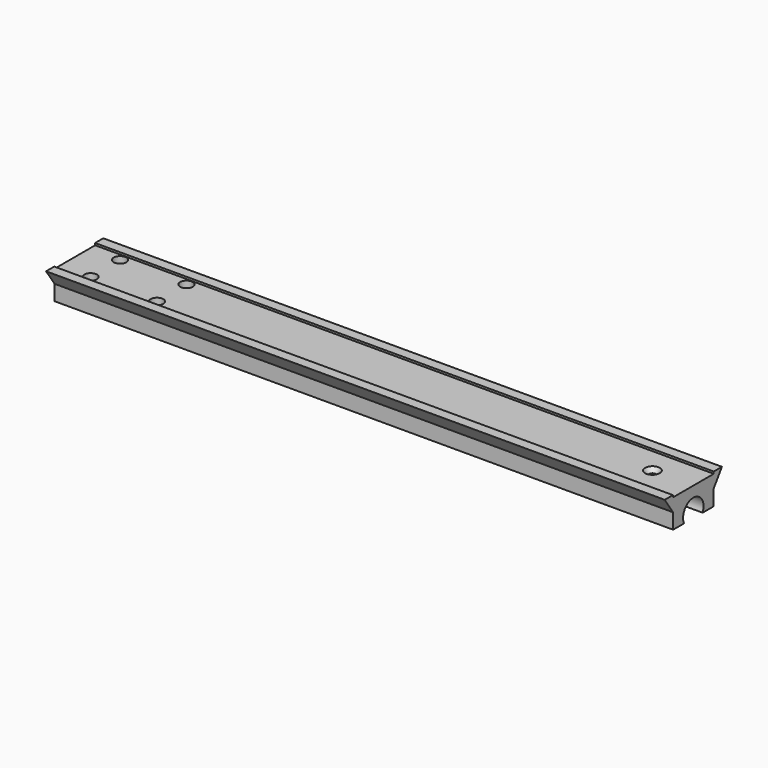
from build123d import *

# Parameters (mm, degrees)
F5_D           = 4.4958
F5_START       = 1.27
F5_CSINK_D     = 9.1186
F5_CSINK_ANGLE = 82
F9_D           = 5.1054
F9_CBORE_D     = 7.9375
F9_CBORE_DEPTH = 4.826


# Not quite as in the source:
# - a feature names something its author has since deleted; it is built from what else it names


with BuildPart() as f2:
    # F2: sweep along a path in F0
    with BuildLine(Plane.XZ) as f2_path:
        Line((384.6068, 55.8292), (0, 55.8292))
    # F1 (on Right) → F2 (sweep)
    with BuildSketch(Plane.YZ):
        with BuildLine():
            Line((15.875, 54.5592), (0, 54.5592))
            Line((0, 54.5592), (-15.875, 54.5592))
            Line((-15.875, 54.5592), (-15.875, 55.8292))
            Line((-15.875, 55.8292), (-22.225, 55.8292))
            Line((-22.225, 55.8292), (-15.6786488693, 46.3042))
            Line((-15.6786488693, 46.3042), (-15.6786488693, 36.7792))
            Line((-15.6786488693, 36.7792), (-7.2411052202, 36.7792))
            ThreePointArc((-7.2411052202, 36.7792), (0, 47.9679), (7.2411052202, 36.7792))
            Line((7.2411052202, 36.7792), (15.6786488693, 36.7792))
            Line((15.6786488693, 36.7792), (15.6786488693, 46.3042))
            Line((15.6786488693, 46.3042), (22.225, 55.8292))
            Line((22.225, 55.8292), (15.875, 55.8292))
            Line((15.875, 55.8292), (15.875, 54.5592))
        make_face()
    sweep(path=f2_path.line)

    # F5 (through all)
    # its depths count from where the whole tool has entered the part; down to there all is cleared
    with Locations(Plane.XY.offset(55.8292).offset(-F5_START)):
        with Locations((359.2068, 0)):
            CounterSinkHole(F5_D / 2, F5_CSINK_D / 2, counter_sink_angle=F5_CSINK_ANGLE)

    # F9 (through all)
    with Locations(Plane.XY.offset(54.5592)):
        with Locations((60.325, 11.4598770448), (60.325, -11.4598770448), (19.05, -11.4598770448), (19.05, 11.4598770448)):
            CounterBoreHole(F9_D / 2, F9_CBORE_D / 2, F9_CBORE_DEPTH)


solid = f2.part
